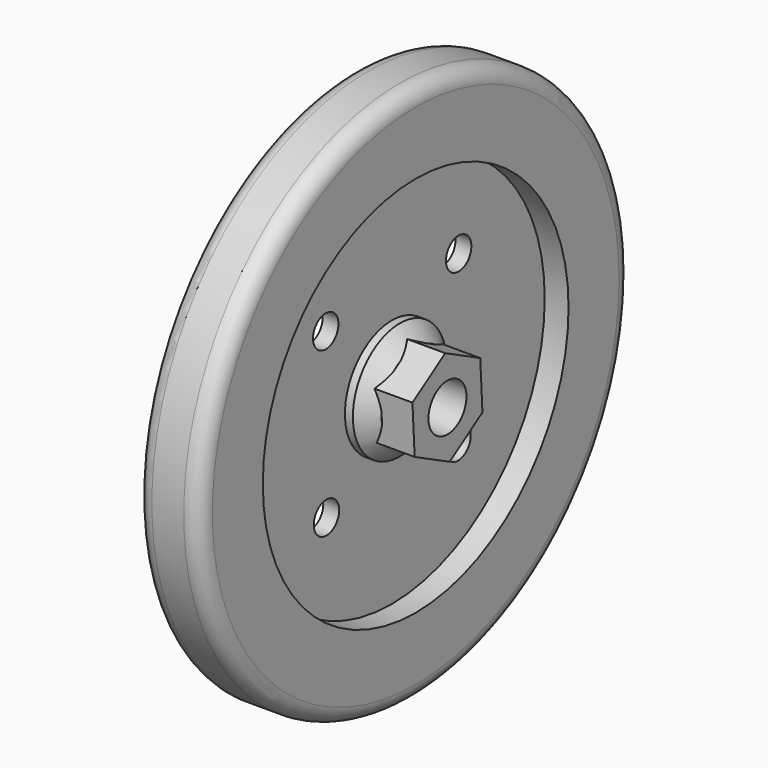
from build123d import *

# Parameters (mm, degrees)
F0_R     = 85
F0_R_2   = 60.1341050947
F1_DEPTH = 10
F0_R_3   = 5
F0_R_4   = 18.4571799951
F2_DEPTH = 2.5
F3_DEPTH = 10
F4_R     = 5
F0_R_5   = 7.4694808043
F6_DEPTH = 20


# Not quite as in the source:
# - a fillet or chamfer that OpenCascade refuses, or shapes differently, is made with other operations: its cross-section is extruded or revolved along the edge and cut away or added


with BuildPart() as f1:
    # F0 (on Right) → F1 (new body, symmetric)
    with BuildSketch(Plane.YZ):
        Circle(F0_R)
        Circle(F0_R_2, mode=Mode.SUBTRACT)
    extrude(amount=F1_DEPTH, both=True)

    # F0 (on Right) → F2 (join, symmetric)
    with BuildSketch(Plane.YZ):
        Circle(F0_R_2)
        with Locations((-25.7258657366, -25.725863874)):
            Circle(F0_R_3, mode=Mode.SUBTRACT)
        with Locations((26.0370634496, -26.0024871677)):
            Circle(F0_R_3, mode=Mode.SUBTRACT)
        with Locations((-26, 26)):
            Circle(F0_R_3, mode=Mode.SUBTRACT)
        Circle(F0_R_4, mode=Mode.SUBTRACT)
        with Locations((26.2791067362, 26.2791085988)):
            Circle(F0_R_3, mode=Mode.SUBTRACT)
    extrude(amount=F2_DEPTH, both=True)

    # F0 (on Right) → F3 (join, symmetric)
    with BuildSketch(Plane.YZ):
        Circle(F0_R_4)
        Polygon((12.8988242803, 8.4499999602), (13.7673267676, -6.9457095256), (0.8685024874, -15.3957094858), (-12.8988242803, -8.4499999602), (-13.7673267676, 6.9457095256), (-0.8685024874, 15.3957094858), align=None, mode=Mode.SUBTRACT)
    extrude(amount=F3_DEPTH, both=True)

    # F4
    f4_edges = [f1.edges().sort_by_distance(p)[0] for p in [
        (-10, -85, 0),
        (10, -85, 0),
    ]]
    fillet(f4_edges, radius=F4_R)

    # F5: chamfer of 5 on 2 edges, made by hand

    # F5_s1 → F5_t2 (revolve, cut)
    with BuildSketch(Plane.XY):
        Polygon((5, 18.4571799951), (10, 13.4571799951), (10, 18.4571799951), align=None)
    revolve(axis=Axis((10, 0, 0), (1, 0, 0)), mode=Mode.SUBTRACT)

    # F5_s3 → F5_t4 (revolve, cut)
    with BuildSketch(Plane.XY):
        Polygon((-5, 18.4571799951), (-10, 13.4571799951), (-10, 18.4571799951), align=None)
    revolve(axis=Axis((-10, 0, 0), (1, 0, 0)), mode=Mode.SUBTRACT)

    # F0 (on Right) → F6 (join)
    with BuildSketch(Plane.YZ):
        Polygon((0.8685024874, -15.3957094858), (13.7673267676, -6.9457095256), (12.8988242803, 8.4499999602), (-0.8685024874, 15.3957094858), (-13.7673267676, 6.9457095256), (-12.8988242803, -8.4499999602), align=None)
        Circle(F0_R_5, mode=Mode.SUBTRACT)
    extrude(amount=F6_DEPTH)


solid = f1.part
